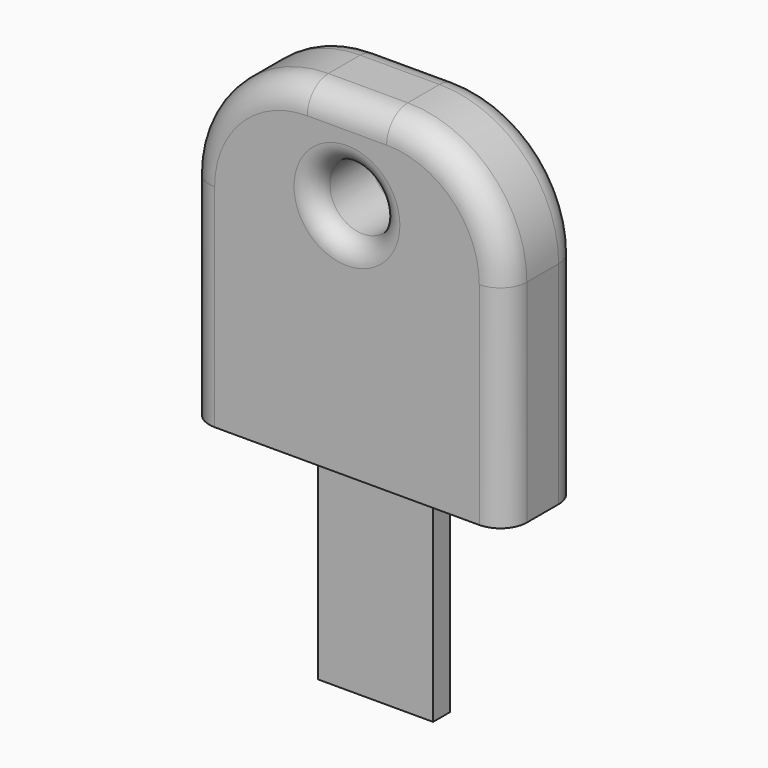
from build123d import *

# Parameters (mm, degrees)
F0_W         = 24
F0_H         = 25
F1_DEPTH     = 3.5
F2_R         = 2
F4_DEPTH     = 0.8
F5_R         = 2.5
F6_DEPTH     = 7.001
F8_R         = 1.5
F9_T1_DEPTH  = 7
F9_T4_ANGLE  = 90
F9_T6_ANGLE  = 90
F9_T8_ANGLE  = 90
F9_T10_ANGLE = 90


# Not quite as in the source:
# - a fillet or chamfer that OpenCascade refuses, or shapes differently, is made with other operations: its cross-section is extruded or revolved along the edge and cut away or added


with BuildPart() as f1:
    # F0 (on Front) → F1 (new body, symmetric)
    with BuildSketch(Plane.XZ):
        with Locations((0, 12.5)):
            Rectangle(F0_W, F0_H)
    extrude(amount=F1_DEPTH, both=True)

    # F2
    f2_edges = [f1.edges().sort_by_distance(p)[0] for p in [
        (0, -3.5, 25),
        (0, 3.5, 25),
        (-12, -3.5, 12.5),
        (-12, 3.5, 12.5),
        (12, -3.5, 12.5),
        (12, 3.5, 12.5),
    ]]
    fillet(f2_edges, radius=F2_R)

    # F5 (on face) → F6 (cut, through all)
    with BuildSketch(Plane.XZ.offset(3.5)):
        with Locations((0, 18)):
            Circle(F5_R)
    extrude(amount=-F6_DEPTH, mode=Mode.SUBTRACT)


with BuildPart() as f4:
    # F3 (on Front) → F4 (new body, symmetric)
    with BuildSketch(Plane.XZ):
        with BuildLine():
            Line((-4.35, 8.5), (-4.35, 5.4))
            ThreePointArc((-4.35, 5.4), (-3.75, 3.9), (-4.35, 2.4))
            Line((-4.35, 2.4), (-4.35, -16.0384941622))
            Line((-4.35, -16.0384941622), (4.35, -16.0384941622))
            Line((4.35, -16.0384941622), (4.35, 2.4))
            ThreePointArc((4.35, 2.4), (3.75, 3.9), (4.35, 5.4))
            Line((4.35, 5.4), (4.35, 8.5))
            Line((4.35, 8.5), (2.05, 8.5))
            Line((2.05, 8.5), (2.05, 4.55))
            ThreePointArc((2.05, 4.55), (0, 2.5), (-2.05, 4.55))
            Line((-2.05, 4.55), (-2.05, 8.5))
            Line((-2.05, 8.5), (-4.35, 8.5))
        make_face()
    extrude(amount=F4_DEPTH, both=True)


with BuildPart() as f1_1:
    add(f1.part)

    # F7: cut F4
    add(f4.part, mode=Mode.SUBTRACT)

    # F8
    f8_edges = [f1_1.edges().sort_by_distance(p)[0] for p in [
        (-2.5, 3.5, 18),
        (-2.5, -3.5, 18),
    ]]
    fillet(f8_edges, radius=F8_R)

    # F9: fillet of radius 9 on 2 edges, made by hand

    # F9_s2 → F9_t1 (cut)
    with BuildSketch(Plane.XZ.offset(-3.5)):
        with BuildLine():
            ThreePointArc((12, 16), (9.3639610307, 22.3639610307), (3, 25))
            Line((3, 25), (12, 25))
            Line((12, 25), (12, 16))
        make_face()
        with BuildLine():
            ThreePointArc((-12, 16), (-9.3639610307, 22.3639610307), (-3, 25))
            Line((-3, 25), (-12, 25))
            Line((-12, 25), (-12, 16))
        make_face()
    extrude(amount=F9_T1_DEPTH, mode=Mode.SUBTRACT)

    # F9_s3 → F9_t4 (revolve, cut)
    with BuildSketch(Plane.XY.offset(16)):
        with BuildLine():
            ThreePointArc((-10, 3.5), (-11.4142135624, 2.9142135624), (-12, 1.5))
            Line((-12, 1.5), (-12, 3.5))
            Line((-12, 3.5), (-10, 3.5))
        make_face()
    revolve(axis=Axis((-3, 3.5, 16), (0, 1, 0)), revolution_arc=F9_T4_ANGLE, mode=Mode.SUBTRACT)

    # F9_s5 → F9_t6 (revolve, cut)
    with BuildSketch(Plane.YZ.offset(-3)):
        with BuildLine():
            ThreePointArc((-3.5, 23), (-2.9142135624, 24.4142135624), (-1.5, 25))
            Line((-1.5, 25), (-3.5, 25))
            Line((-3.5, 25), (-3.5, 23))
        make_face()
    revolve(axis=Axis((-3, -3.5, 16), (0, -1, 0)), revolution_arc=F9_T6_ANGLE, mode=Mode.SUBTRACT)

    # F9_s7 → F9_t8 (revolve, cut)
    with BuildSketch(Plane.XY.offset(16)):
        with BuildLine():
            ThreePointArc((10, -3.5), (11.4142135624, -2.9142135624), (12, -1.5))
            Line((12, -1.5), (12, -3.5))
            Line((12, -3.5), (10, -3.5))
        make_face()
    revolve(axis=Axis((3, -3.5, 16), (0, -1, 0)), revolution_arc=F9_T8_ANGLE, mode=Mode.SUBTRACT)

    # F9_s9 → F9_t10 (revolve, cut)
    with BuildSketch(Plane.YZ.offset(3)):
        with BuildLine():
            ThreePointArc((3.5, 23), (2.9142135624, 24.4142135624), (1.5, 25))
            Line((1.5, 25), (3.5, 25))
            Line((3.5, 25), (3.5, 23))
        make_face()
    revolve(axis=Axis((3, 3.5, 16), (0, 1, 0)), revolution_arc=F9_T10_ANGLE, mode=Mode.SUBTRACT)


solid = Compound([f4.part, f1_1.part])
